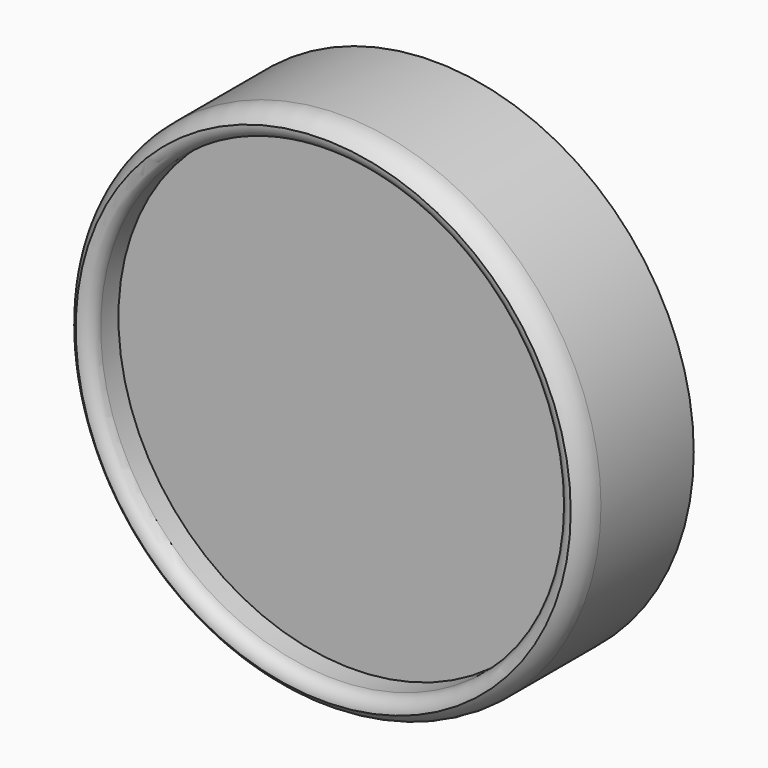
from build123d import *

# Parameters (mm, degrees)
F0_R     = 47.4803675011
F0_R_2   = 42.7485217124
F1_DEPTH = 25.4
F2_DEPTH = 18.796
F3_R     = 2.54


# Not quite as in the source:
# - a fillet or chamfer that OpenCascade refuses, or shapes differently, is made with other operations: its cross-section is extruded or revolved along the edge and cut away or added


with BuildPart() as f1:
    # F0 (on Front) → F1 (new body)
    with BuildSketch(Plane.XZ):
        Circle(F0_R)
        Circle(F0_R_2, mode=Mode.SUBTRACT)
    extrude(amount=F1_DEPTH)

    # F0 (on Front) → F2 (join)
    with BuildSketch(Plane.XZ):
        Circle(F0_R_2)
    extrude(amount=F2_DEPTH)

    # F3
    f3_edges = [f1.edges().sort_by_distance(p)[0] for p in [
        (-42.748522, -25.4, 0),
    ]]
    fillet(f3_edges, radius=F3_R)

    # F4: fillet of radius 5.08 on 1 edges, made by hand

    # F4_s1 → F4_t2 (revolve, cut)
    with BuildSketch(Plane.XY):
        with BuildLine():
            ThreePointArc((45.2885217124, -25.4), (46.8991575269, -23.5803996015), (47.4803675011, -21.2208894186))
            Line((47.4803675011, -21.2208894186), (47.4803675011, -25.4))
            Line((47.4803675011, -25.4), (45.2885217124, -25.4))
        make_face()
    revolve(axis=Axis((0, -25.4, 0), (0, -1, 0)), mode=Mode.SUBTRACT)


solid = f1.part
